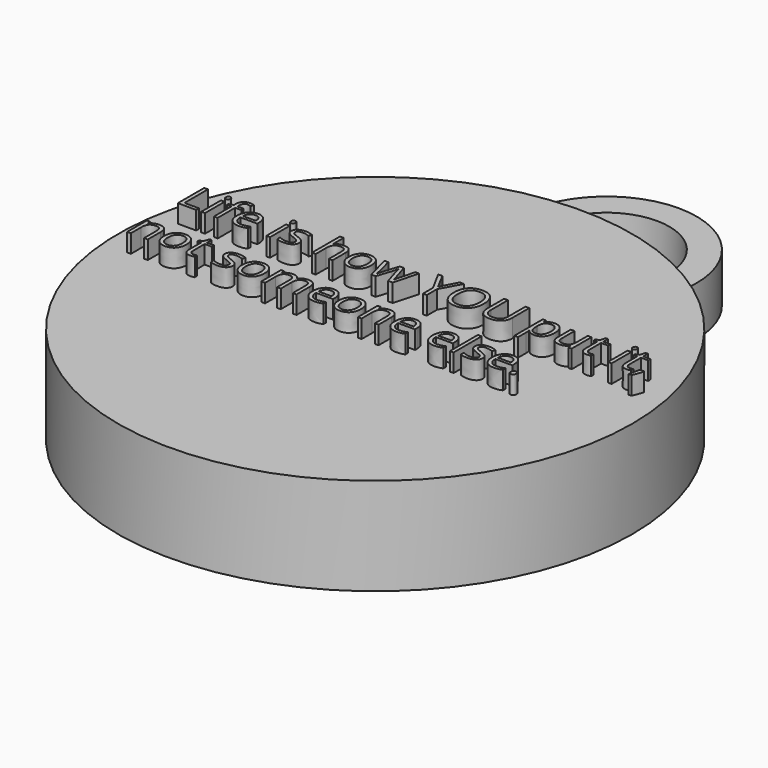
from build123d import *

# Parameters (mm, degrees)
F0_R         = 50.3789129072
F1_DEPTH     = 19.05
F2_TEXT_SIZE = 9.0313603222
F3_DEPTH     = 3.556
F4_R         = 17.6632657844
F4_R_2       = 12.2951036427
F5_DEPTH     = 9.652


# Not quite as in the source:
# - Text() gives the source's letters only with a copy of the font that has no kerning and outlines rounded to 1/6400 em; it was checked with that copy


with BuildPart() as f1:
    # F0 (on Top) → F1 (new body)
    with BuildSketch(Plane.XY):
        Circle(F0_R)
    extrude(amount=F1_DEPTH)

    # F2 (on face) → F3 (join)
    with BuildSketch(Plane.XY.offset(19.05)):
        with Locations((-46.2248618715, 8.3402651362)):
            Text('Life is how YOU put it,', F2_TEXT_SIZE, font='Open Sans', text_align=(TextAlign.LEFT, TextAlign.BOTTOM))
        with Locations((-46.2248618715, -3.942384902)):
            Text('not someone else.', F2_TEXT_SIZE, font='Open Sans', text_align=(TextAlign.LEFT, TextAlign.BOTTOM))
    extrude(amount=F3_DEPTH)

    # F4 (on Top) → F5 (join)
    with BuildSketch(Plane.XY):
        with Locations((0, 56.6855296493)):
            Circle(F4_R)
        with Locations((0, 56.6855296493)):
            Circle(F4_R_2, mode=Mode.SUBTRACT)
    extrude(amount=F5_DEPTH)


solid = f1.part
